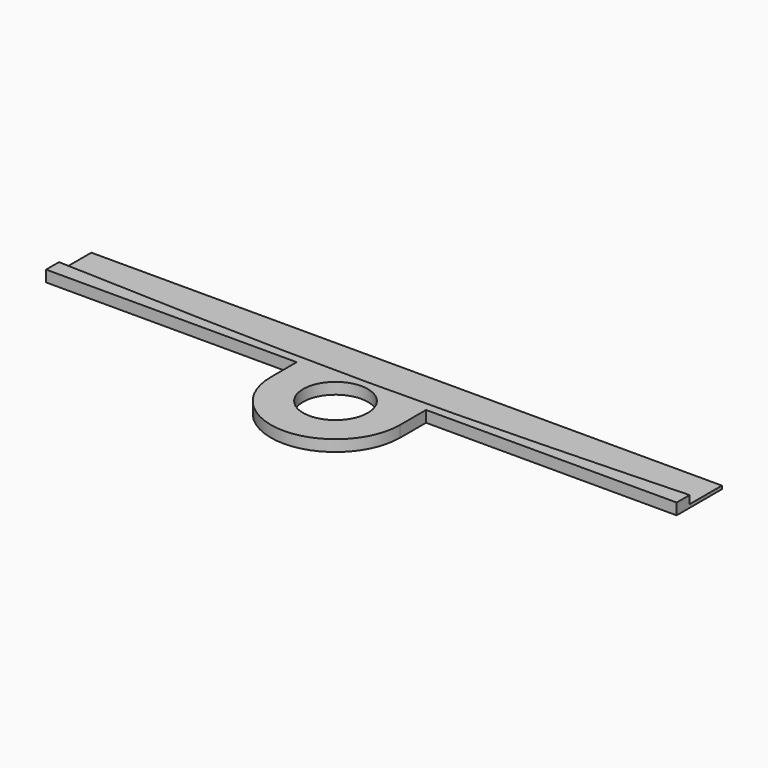
from build123d import *

# Parameters (mm, degrees)
F0_W      = 97.5
F0_H      = 15
F1_DEPTH  = 1
F2_W      = 77.5
F2_H      = 2.5
F3_DEPTH  = 3.5
F4_DEPTH  = 3.5
F5_R      = 10
F7_DEPTH  = 3.5
F10_DEPTH = 3.5


# Not quite as in the source:
# - a feature of the source that left no trace in its solid (it failed there, or was rolled back) is left out
# - a feature names something its author has since deleted; it is built from what else it names


with BuildPart() as f1:
    # F0 (on Top) → F1 (new body)
    with BuildSketch(Plane.XY):
        with Locations((-48.75, 7.5)):
            Rectangle(F0_W, F0_H)
        with Locations((48.75, 7.5)):
            Rectangle(F0_W, F0_H)
    extrude(amount=F1_DEPTH)

    # F2 (on Top) → F3 (join)
    with BuildSketch(Plane.XY):
        with Locations((58.75, -1.25)):
            Rectangle(F2_W, F2_H)
        with Locations((-58.75, -1.25)):
            Rectangle(F2_W, F2_H)
        with BuildLine():
            ThreePointArc((-17.3205080757, -2.5), (-16.5138781887, -1.2176320229), (-15.612494996, 0))
            Line((-15.612494996, 0), (-20, 0))
            Line((-20, 0), (-20, -2.5))
            Line((-20, -2.5), (-17.3205080757, -2.5))
        make_face()
        with BuildLine():
            ThreePointArc((-20, -12.5), (-19.3185165258, -7.3236190979), (-17.3205080757, -2.5))
            Line((-17.3205080757, -2.5), (-20, -2.5))
            Line((-20, -2.5), (-20, -12.5))
        make_face()
        with BuildLine():
            Line((20, 0), (15.612494996, 0))
            ThreePointArc((15.612494996, 0), (16.5138781887, -1.2176320229), (17.3205080757, -2.5))
            Line((17.3205080757, -2.5), (20, -2.5))
            Line((20, -2.5), (20, 0))
        make_face()
        with BuildLine():
            Line((20, -2.5), (17.3205080757, -2.5))
            ThreePointArc((17.3205080757, -2.5), (19.3185165258, -7.3236190979), (20, -12.5))
            Line((20, -12.5), (20, -2.5))
        make_face()
    extrude(amount=F3_DEPTH)

    # F2 (on Top) → F4 (join)
    with BuildSketch(Plane.XY):
        with BuildLine():
            Line((15.612494996, 0), (0, 0))
            Line((0, 0), (-15.612494996, 0))
            ThreePointArc((-15.612494996, 0), (-16.5138781887, -1.2176320229), (-17.3205080757, -2.5))
            Line((-17.3205080757, -2.5), (17.3205080757, -2.5))
            ThreePointArc((17.3205080757, -2.5), (16.5138781887, -1.2176320229), (15.612494996, 0))
        make_face()
        with BuildLine():
            ThreePointArc((20, -12.5), (19.3185165258, -7.3236190979), (17.3205080757, -2.5))
            Line((17.3205080757, -2.5), (-17.3205080757, -2.5))
            ThreePointArc((-17.3205080757, -2.5), (-19.3185165258, -7.3236190979), (-20, -12.5))
            Line((-20, -12.5), (20, -12.5))
        make_face()
        with BuildLine():
            ThreePointArc((-20, -12.5), (0, -32.5), (20, -12.5))
            Line((20, -12.5), (-20, -12.5))
        make_face()
    extrude(amount=F4_DEPTH)

    # F6: union 

    # F5 (on face) → F7 (cut)
    with BuildSketch(Plane.XY.offset(3.5)):
        with Locations((0, -12.5)):
            Circle(F5_R)
    extrude(amount=-F7_DEPTH, mode=Mode.SUBTRACT)

    # F8 (on face) → F10 (join)
    with BuildSketch(Plane.XY.offset(3.5)):
        with BuildLine():
            add(Edge.make_bspline(
                [(-97.5, 2.5), (-65, 1.25), (-32.5, 0), (0, 0)],
                knots=[0, 0, 0, 0, 0.5, 0.5, 0.5, 0.5], degree=3))
            Line((-97.5, 2.5), (-97.5, 0))
            Line((-97.5, 0), (0, 0))
        make_face()
        with BuildLine():
            add(Edge.make_bspline(
                [(0, 0), (32.5, 0), (65, 1.25), (97.5, 2.5)],
                knots=[0.5, 0.5, 0.5, 0.5, 1, 1, 1, 1], degree=3))
            Line((0, 0), (97.5, 0))
            Line((97.5, 0), (97.5, 2.5))
        make_face()
    extrude(amount=-F10_DEPTH)


solid = f1.part
